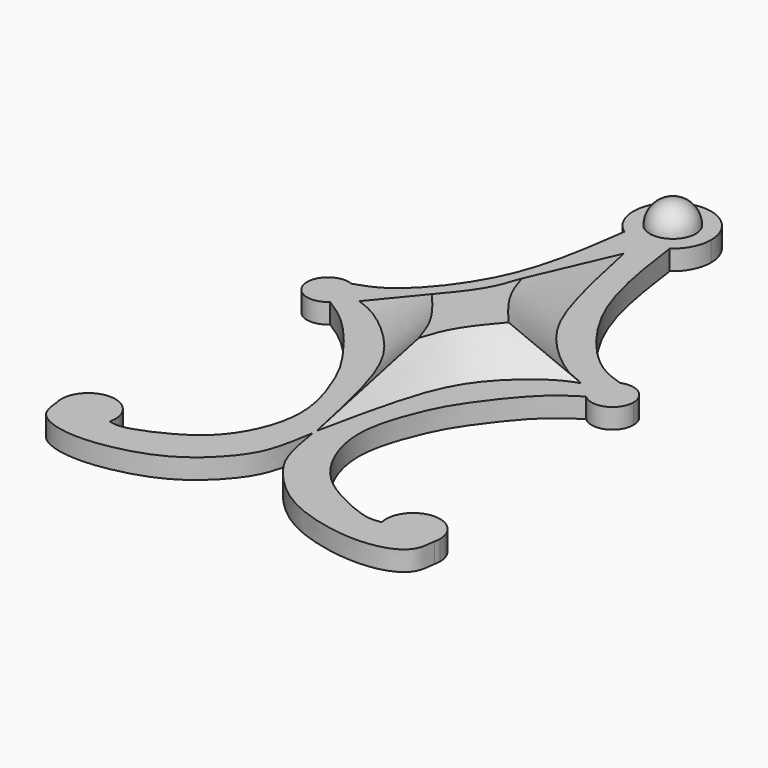
from build123d import *

# Parameters (mm, degrees)
F1_DEPTH = 2


with BuildPart() as f1:
    # F0 (on Top) → F1 (new body)
    with BuildSketch(Plane.XY):
        with BuildLine():
            ThreePointArc((2.276998472, 22.1518947859), (3.4684353098, 23.5377967667), (3.8970014846, 25.3144726157))
            ThreePointArc((3.8970014846, 25.3144726157), (-1.776675849, 28.7829079255), (-2.276998472, 22.1518947859))
            ThreePointArc((-2.276998472, 22.1518947859), (0, 21.4174711311), (2.276998472, 22.1518947859))
        make_face()
        with BuildLine():
            ThreePointArc((2.276998472, 22.1518947859), (0, 21.4174711311), (-2.276998472, 22.1518947859))
            add(Edge.make_bspline(
                [(-2.276998472, 22.1518947859), (-2.43209236, 20.9439660702), (-2.8343734971, 18.0367414787), (-4.2933644234, 10.5944689547), (-8.8445045466, 4.3730220087), (-11.8033781804, 2.4111709095), (-13.0773430388, 2.1147085966), (-13.4704228381, 1.9336606815)],
                knots=[0, 0, 0, 0, 0.1881889821, 0.4481491748, 0.7093502782, 0.8822992894, 1, 1, 1, 1], degree=3))
            ThreePointArc((-13.4704228381, 1.9336606815), (-12.5293900739, 1.1634963246), (-12.1758761383, 0))
            ThreePointArc((-12.1758761383, 0), (-12.3466918638, -0.827839696), (-12.831236523, -1.520452898))
            add(Edge.make_bspline(
                [(-12.831236523, -1.520452898), (-11.8842823807, -2.1213598077), (-9.681883743, -3.5201856027), (-5.5850911002, -8.9136286048), (-4.2143400839, -11.8630451312), (-2.0601001418, -17.7294924846), (-4.5364296122, -24.1123047819), (-8.3995913538, -26.8506466614), (-12.2431889954, -28.4193492404), (-13.2719842293, -28.2231302019), (-13.6472955259, -28.1513297683)],
                knots=[0, 0, 0, 0, 0.116209539, 0.2700802769, 0.3818783209, 0.5275533776, 0.680317664, 0.8123481439, 0.9316634476, 1, 1, 1, 1], degree=3))
            ThreePointArc((-13.6472955259, -28.1513297683), (-16.2800811231, -30.2281833728), (-18.9128667203, -28.1513297683))
            add(Edge.make_bspline(
                [(-18.9128667203, -28.1513297683), (-18.8376863203, -28.9308803678), (-18.6694510212, -30.675323445), (-14.9675114924, -32.0694588166), (-9.6030872532, -31.3634199504), (-5.1754016498, -29.5295339957), (-1.8867493119, -26.1259118959), (-0.6530666103, -23.5893108184), (-0.2293292758, -21.1004769068), (0, -19.7535045445)],
                knots=[0, 0, 0, 0, 0.1097624217, 0.2456213834, 0.4165331309, 0.578325558, 0.7339136873, 0.8559924358, 1, 1, 1, 1], degree=3))
            add(Edge.make_bspline(
                [(18.9128667203, -28.1513297683), (18.8376863203, -28.9308803678), (18.6694510212, -30.675323445), (14.9675114924, -32.0694588166), (9.6030872532, -31.3634199504), (5.1754016498, -29.5295339957), (1.8867493119, -26.1259118959), (0.6530666103, -23.5893108184), (0.2293292758, -21.1004769068), (0, -19.7535045445)],
                knots=[0, 0, 0, 0, 0.1097624217, 0.2456213834, 0.4165331309, 0.578325558, 0.7339136873, 0.8559924358, 1, 1, 1, 1], degree=3))
            ThreePointArc((18.9128667203, -28.1513297683), (16.2800811231, -30.2281833728), (13.6472955259, -28.1513297683))
            add(Edge.make_bspline(
                [(12.831236523, -1.520452898), (11.8842823807, -2.1213598077), (9.681883743, -3.5201856027), (5.5850911002, -8.9136286048), (4.2143400839, -11.8630451312), (2.0601001418, -17.7294924846), (4.5364296122, -24.1123047819), (8.3995913538, -26.8506466614), (12.2431889954, -28.4193492404), (13.2719842293, -28.2231302019), (13.6472955259, -28.1513297683)],
                knots=[0, 0, 0, 0, 0.116209539, 0.2700802769, 0.3818783209, 0.5275533776, 0.680317664, 0.8123481439, 0.9316634476, 1, 1, 1, 1], degree=3))
            ThreePointArc((12.831236523, -1.520452898), (12.2107910898, 0.3805587398), (13.4704228381, 1.9336606815))
            add(Edge.make_bspline(
                [(2.276998472, 22.1518947859), (2.43209236, 20.9439660702), (2.8343734971, 18.0367414787), (4.2933644234, 10.5944689547), (8.8445045466, 4.3730220087), (11.8033781804, 2.4111709095), (13.0773430388, 2.1147085966), (13.4704228381, 1.9336606815)],
                knots=[0, 0, 0, 0, 0.1881889821, 0.4481491748, 0.7093502782, 0.8822992894, 1, 1, 1, 1], degree=3))
        make_face()
        with BuildLine():
            ThreePointArc((-12.1758761383, 0), (-12.5293900739, 1.1634963246), (-13.4704228381, 1.9336606815))
            ThreePointArc((-13.4704228381, 1.9336606815), (-16.3238112841, -0.3805587398), (-12.831236523, -1.520452898))
            ThreePointArc((-12.831236523, -1.520452898), (-12.3466918638, -0.827839696), (-12.1758761383, 0))
        make_face()
        with BuildLine():
            ThreePointArc((16.3587262356, 0), (15.4307975115, 1.737911113), (13.4704228381, 1.9336606815))
            ThreePointArc((13.4704228381, 1.9336606815), (12.2107910898, 0.3805587398), (12.831236523, -1.520452898))
            ThreePointArc((12.831236523, -1.520452898), (15.0951408829, -1.9206093231), (16.3587262356, 0))
        make_face()
        with BuildLine():
            ThreePointArc((-18.9128667203, -28.1513297683), (-16.2800811231, -30.2281833728), (-13.6472955259, -28.1513297683))
            ThreePointArc((-13.6472955259, -28.1513297683), (-13.5915554401, -27.8383489621), (-13.5728896121, -27.5209918618))
            ThreePointArc((-13.5728896121, -27.5209918618), (-16.5974382234, -24.8324661788), (-18.9128667203, -28.1513297683))
        make_face()
        with BuildLine():
            ThreePointArc((18.9872726341, -27.5209918618), (15.9627240228, -24.8324661788), (13.6472955259, -28.1513297683))
            ThreePointArc((13.6472955259, -28.1513297683), (16.2800811231, -30.2281833728), (18.9128667203, -28.1513297683))
            ThreePointArc((18.9128667203, -28.1513297683), (18.9686068061, -27.8383489621), (18.9872726341, -27.5209918618))
        make_face()
    extrude(amount=F1_DEPTH)

    # F2 (on face) → F5 section 0
    with BuildSketch(Plane.XY.offset(2)):
        with BuildLine():
            add(Edge.make_bspline(
                [(0, 19.2468184978), (0.6301650981, 16.2510379584), (1.7928287138, 10.723780032), (4.0098790345, 4.9325918727), (8.7986333903, 0.8351177225), (10.4822360359, 0.2324566501), (11.1316302791, 0)],
                knots=[0, 0, 0, 0, 0.3137777977, 0.578924523, 0.8375840098, 1, 1, 1, 1], degree=3))
            add(Edge.make_bspline(
                [(0, 19.2468184978), (-0.6301650981, 16.2510379584), (-1.7928287138, 10.723780032), (-4.0098790345, 4.9325918727), (-8.7986333903, 0.8351177225), (-10.4822360359, 0.2324566501), (-11.1316302791, 0)],
                knots=[0, 0, 0, 0, 0.3137777977, 0.578924523, 0.8375840098, 1, 1, 1, 1], degree=3))
            add(Edge.make_bspline(
                [(0, -19.2468184978), (-0.6301650981, -16.2510379584), (-1.7928287138, -10.723780032), (-4.0098790345, -4.9325918727), (-8.7986333903, -0.8351177225), (-10.4822360359, -0.2324566501), (-11.1316302791, 0)],
                knots=[0, 0, 0, 0, 0.3137777977, 0.578924523, 0.8375840098, 1, 1, 1, 1], degree=3))
            add(Edge.make_bspline(
                [(0, -19.2468184978), (0.6301650981, -16.2510379584), (1.7928287138, -10.723780032), (4.0098790345, -4.9325918727), (8.7986333903, -0.8351177225), (10.4822360359, -0.2324566501), (11.1316302791, 0)],
                knots=[0, 0, 0, 0, 0.3137777977, 0.578924523, 0.8375840098, 1, 1, 1, 1], degree=3))
        make_face()
    # F4 (on offset) → F5 section 1
    with BuildSketch(Plane.XY.offset(5)):
        with BuildLine():
            add(Edge.make_bspline(
                [(0, 6.4514661208), (0.2840723178, 5.5826456273), (0.851655844, 3.8467207648), (2.4773384631, 1.6062376793), (3.4071339479, 0.5107520935), (3.8406357635, 0)],
                knots=[0, 0, 0, 0, 0.3484590253, 0.6962297623, 1, 1, 1, 1], degree=3))
            add(Edge.make_bspline(
                [(0, 6.4514661208), (-0.2840723178, 5.5826456273), (-0.851655844, 3.8467207648), (-2.4773384631, 1.6062376793), (-3.4071339479, 0.5107520935), (-3.8406357635, 0)],
                knots=[0, 0, 0, 0, 0.3484590253, 0.6962297623, 1, 1, 1, 1], degree=3))
            add(Edge.make_bspline(
                [(0, -6.4514661208), (-0.2840723178, -5.5826456273), (-0.851655844, -3.8467207648), (-2.4773384631, -1.6062376793), (-3.4071339479, -0.5107520935), (-3.8406357635, 0)],
                knots=[0, 0, 0, 0, 0.3484590253, 0.6962297623, 1, 1, 1, 1], degree=3))
            add(Edge.make_bspline(
                [(0, -6.4514661208), (0.2840723178, -5.5826456273), (0.851655844, -3.8467207648), (2.4773384631, -1.6062376793), (3.4071339479, -0.5107520935), (3.8406357635, 0)],
                knots=[0, 0, 0, 0, 0.3484590253, 0.6962297623, 1, 1, 1, 1], degree=3))
        make_face()
    loft()

    # F6 (on face) → F7 (revolve)
    with BuildSketch(Plane.XY.offset(2)):
        with BuildLine():
            Line((0, 23.0819760401), (0, 27.6924492281))
            ThreePointArc((0, 27.6924492281), (-2.305236594, 25.3872126341), (0, 23.0819760401))
        make_face()
    revolve(axis=Axis((0, 25.3872126341, 2), (0, -1, 0)))


solid = f1.part
